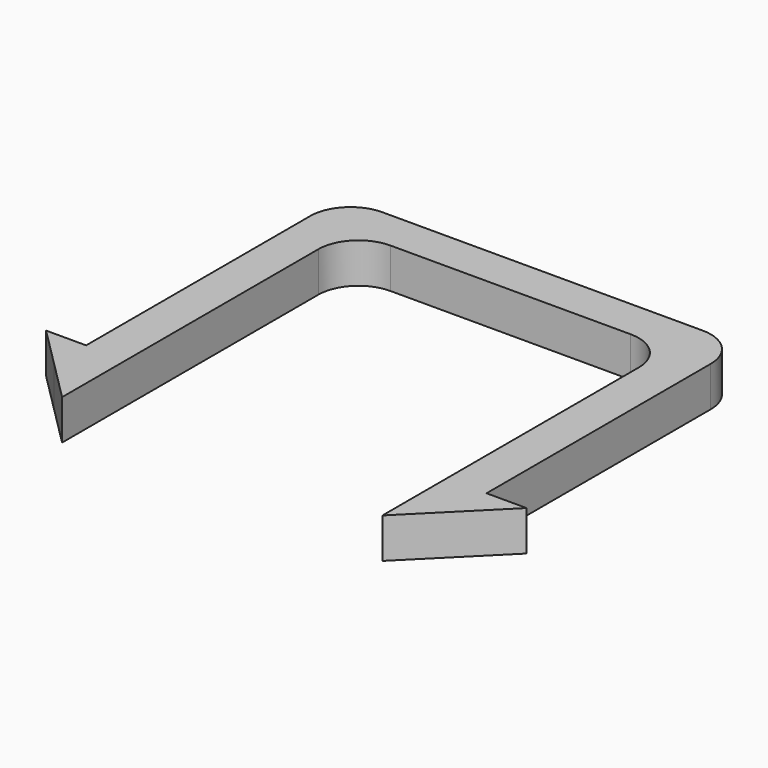
from build123d import *

# Parameters (mm, degrees)
F0_W      = 50
F0_H      = 50
F1_DEPTH  = 5
F2_W      = 40
F2_H      = 45
F3_DEPTH  = 5.001
F4_R      = 5
F6_DEPTH  = 5
F8_DEPTH  = 5.001
F10_DEPTH = 5
F12_DEPTH = 5.001


# Not quite as in the source:
# - ends of sketch curves that miss each other by under 0.0002 mm in the source are joined


with BuildPart() as f1:
    # F0 (on Top) → F1 (new body)
    with BuildSketch(Plane.XY):
        Rectangle(F0_W, F0_H)
    extrude(amount=F1_DEPTH)

    # F2 (on face) → F3 (cut, through all)
    with BuildSketch(Plane.XY.offset(5)):
        with Locations((0, -2.5)):
            Rectangle(F2_W, F2_H)
    extrude(amount=-F3_DEPTH, mode=Mode.SUBTRACT)

    # F4
    f4_edges = [f1.edges().sort_by_distance(p)[0] for p in [
        (-20, 20, 2.5),
        (20, 20, 2.5),
        (25, 25, 2.5),
        (-25, 25, 2.5),
    ]]
    fillet(f4_edges, radius=F4_R)

    # F5 (on face) → F6 (join)
    with BuildSketch(Plane.XY.offset(5)):
        Polygon((-25, -19.9999040991), (-25, -15), (-30, -15), align=None)
    extrude(amount=-F6_DEPTH)

    # F7 (on face) → F8 (cut, through all)
    with BuildSketch(Plane.XY.offset(5)):
        Polygon((-20, -25), (-25.0000479505, -19.9999520495), (-25, -25), align=None)
    extrude(amount=-F8_DEPTH, mode=Mode.SUBTRACT)

    # F9 (on Top) → F10 (join)
    with BuildSketch(Plane.XY):
        Polygon((30, -15), (25, -15), (25, -20), align=None)
    extrude(amount=F10_DEPTH)

    # F11 (on face) → F12 (cut, through all)
    with BuildSketch(Plane.XY.offset(5)):
        Polygon((25, -25), (25, -20), (20, -25), align=None)
    extrude(amount=-F12_DEPTH, mode=Mode.SUBTRACT)


solid = f1.part
